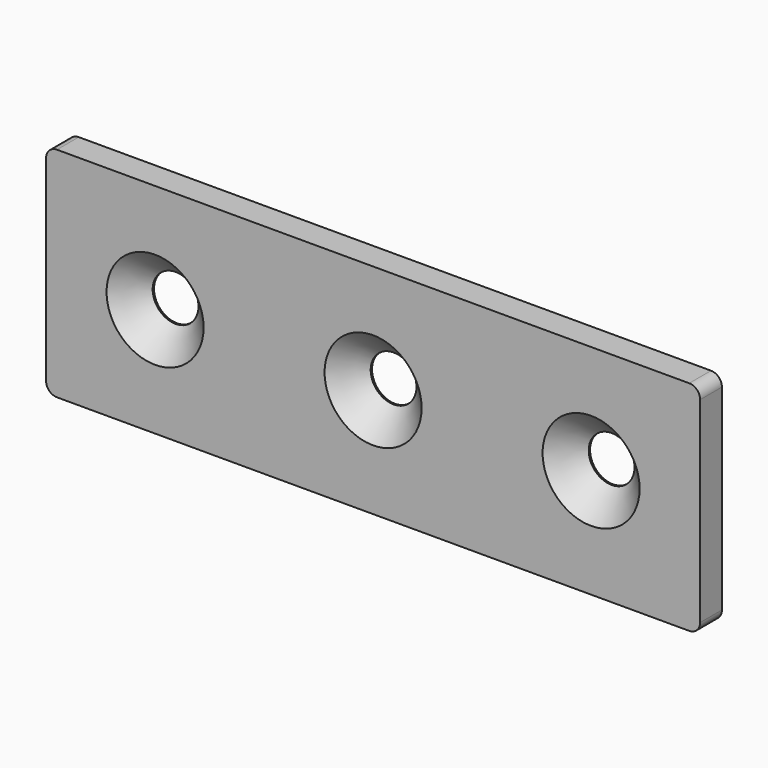
from build123d import *

# Parameters (mm, degrees)
F0_R     = 4.2
F1_DEPTH = 5
F2_SIZE  = 4.7


# Not quite as in the source:
# - a feature names something its author has since deleted; it is built from what else it names


with BuildPart() as f1:
    # F0 (on Front) → F1 (new body)
    with BuildSketch(Plane.XZ):
        with BuildLine():
            Line((98, 20), (-18, 20))
            ThreePointArc((-18, 20), (-19.4142135624, 19.4142135624), (-20, 18))
            Line((-20, 18), (-20, -18))
            ThreePointArc((-20, -18), (-19.4142135624, -19.4142135624), (-18, -20))
            Line((-18, -20), (98, -20))
            ThreePointArc((98, -20), (99.4142135624, -19.4142135624), (100, -18))
            Line((100, -18), (100, 18))
            ThreePointArc((100, 18), (99.4142135624, 19.4142135624), (98, 20))
        make_face()
        Circle(F0_R, mode=Mode.SUBTRACT)
        with Locations((40, 0)):
            Circle(F0_R, mode=Mode.SUBTRACT)
        with Locations((80, 0)):
            Circle(F0_R, mode=Mode.SUBTRACT)
    extrude(amount=F1_DEPTH)

    # F2
    f2_edges = [f1.edges().sort_by_distance(p)[0] for p in [
        (-4.2, -5, 0),
        (35.8, -5, 0),
        (75.8, -5, 0),
    ]]
    chamfer(f2_edges, length=F2_SIZE)


solid = f1.part
